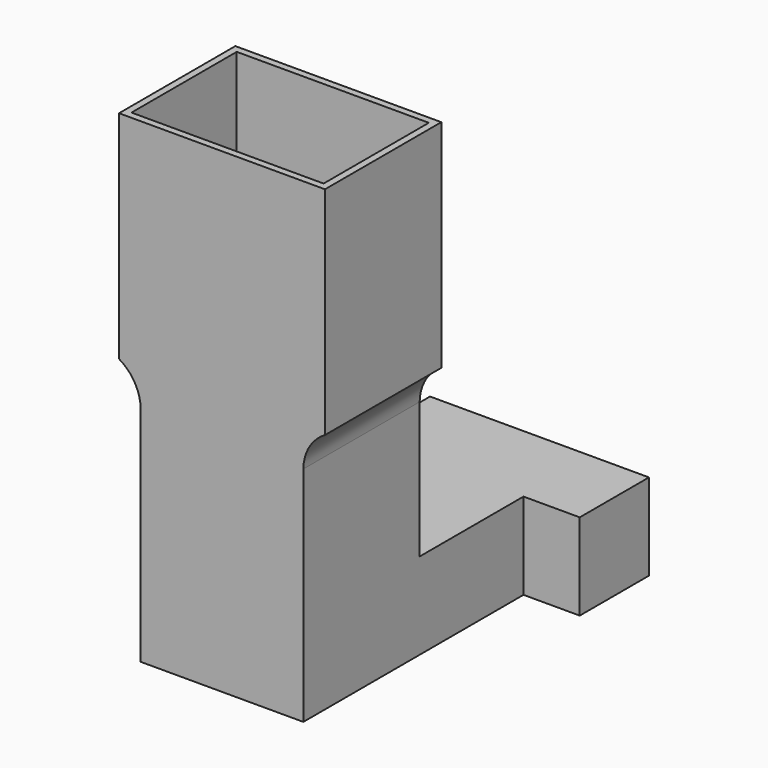
from build123d import *

# Parameters (mm, degrees)
F2_W        = 18.8
F2_H        = 30
F3_DEPTH    = 16.8
F4_T1_DEPTH = 16.8
F5_T        = 0.8
F5_T3_DEPTH = 18.4
F6_W        = 18.8
F6_H        = 10
F7_DEPTH    = 25
F8_T        = -0.8
F9_DEPTH    = 0.8
F10_W       = 0.8
F10_H       = 8.4
F11_DEPTH   = 25.8
F12_W       = 10
F12_H       = 10
F13_DEPTH   = 6.5


# Not quite as in the source:
# - a fillet or chamfer that OpenCascade refuses, or shapes differently, is made with other operations: its cross-section is extruded or revolved along the edge and cut away or added
# - a shell that OpenCascade refuses in one call is made with other operations: the cavity is built on its own and cut out


with BuildPart() as f3:
    # F2 (on Front) → F3 (new body)
    with BuildSketch(Plane.XZ):
        Polygon((23.8, 25), (0, 25), (0, 0), (2.5, 0), (21.3, 0), (23.8, 0), align=None)
        with Locations((11.9, -15)):
            Rectangle(F2_W, F2_H)
    extrude(amount=F3_DEPTH)

    # F4: fillet of radius 5 on 2 edges, made by hand

    # F4_s2 → F4_t1 (join)
    with BuildSketch(Plane.XZ):
        with BuildLine():
            ThreePointArc((0.0002000386, 0.0003463879), (1.8304834454, -1.8302431314), (2.5004, -4.3306845218))
            Line((2.5004, -4.3306845218), (3.0005365685, -4.3306845218))
            ThreePointArc((3.0005365685, -4.3306845218), (3.0001365685, -2.1653422609), (3.0001365685, 0))
            Line((3.0001365685, 0), (2.5, 0.5001365685))
            ThreePointArc((2.5, 0.5001365685), (1.2501000193, 0.5001365685), (0.250316611, 0.4334494788))
            Line((0.250316611, 0.4334494788), (0.0002000386, 0.0003463879))
        make_face()
        with BuildLine():
            ThreePointArc((21.2996, -4.3306845218), (21.9695165546, -1.8302431314), (23.7997999614, 0.0003463879))
            Line((23.7997999614, 0.0003463879), (23.549683389, 0.4334494788))
            ThreePointArc((23.549683389, 0.4334494788), (22.5498999807, 0.5001365685), (21.3, 0.5001365685))
            Line((21.3, 0.5001365685), (20.7998634315, 0))
            ThreePointArc((20.7998634315, 0), (20.7998634315, -2.1653422609), (20.7994634315, -4.3306845218))
            Line((20.7994634315, -4.3306845218), (21.2996, -4.3306845218))
        make_face()
    extrude(amount=F4_T1_DEPTH)

    # F5: shell of thickness 0.8, made by hand


with BuildPart() as f5_core1:
    # F5_t2: copy of F3
    add(f3.part)

    # the walls: a layer under each face that stays
    f5_faces = [f5_core1.faces().sort_by_distance(p)[0] for p in [
        (23.8, -8.4, 12.5),
        (0, -8.4, 12.5),
        (11.9, 0, -2.5),
        (11.9, -16.8, -2.5),
        (23.7996001251, -8.4, 0),
        (0.0003998749, -8.4, 0),
        (21.3, -8.4, -17.1337157982),
        (11.9, -8.4, -30),
        (2.5, -8.4, -17.1337157982),
        (21.9852401758, -8.4, -1.8032011796),
        (1.8147598242, -8.4, -1.8032011796),
    ]]
    thicken(f5_faces, amount=-F5_T, mode=Mode.SUBTRACT)

    # F5_s4 → F5_t3 (cut)
    with BuildSketch(Plane.XZ.offset(-0.8)):
        Polygon((23.803201982, -0.0149272032), (23.7992002503, 0.8), (23.5847337286, 0.8), (23.3990270828, 0.6927203159), align=None)
        Polygon((-0.003201982, -0.0149272032), (0.0007997497, 0.8), (0.2152662714, 0.8), (0.4009729172, 0.6927203159), align=None)
        Polygon((21.3159993602, -4.2675327735), (20.5, -4.2674315965), (20.5, -4.2623725419), (20.5000639825, -4.257313892), align=None)
        Polygon((2.4840006398, -4.2675327735), (3.3, -4.2674315965), (3.3, -4.2623725419), (3.2999360175, -4.257313892), align=None)
    extrude(amount=F5_T3_DEPTH, mode=Mode.SUBTRACT)


with BuildPart() as f3_1:
    add(f3.part)

    # what is left inside the walls is the cavity
    f5_cavity = [f5_core1.part.solids().sort_by_distance(p)[0] for p in [
        (11.9, -15.992, -11.133333),
    ]]
    add(f5_cavity, mode=Mode.SUBTRACT)

    # F6 (on face) → F7 (join)
    with BuildSketch(Plane(origin=(0, 0, 0), x_dir=(-1, 0, 0), z_dir=(0, 1, 0))):
        with Locations((-11.9, -25)):
            Rectangle(F6_W, F6_H)
    extrude(amount=F7_DEPTH)

    # F8
    f8_openings = [f3_1.faces().sort_by_distance(p)[0] for p in [
        (11.9, 25, -25),
    ]]
    offset(amount=F8_T, openings=f8_openings, kind=Kind.INTERSECTION)

    # F9 (cut, through all): a face of the model
    f9_faces = [f3_1.faces().sort_by_distance(p)[0] for p in [
        (11.9, 0, -25),
    ]]
    extrude(f9_faces, amount=-F9_DEPTH, mode=Mode.SUBTRACT)

    # F10 (on face) → F11 (join, through all)
    with BuildSketch(Plane(origin=(0, 25, 0), x_dir=(-1, 0, 0), z_dir=(0, 1, 0))):
        with Locations((-11.9, -25)):
            Rectangle(F10_W, F10_H)
    extrude(amount=-F11_DEPTH)

    # F12 (on face) → F13 (join)
    with BuildSketch(Plane.YZ.offset(21.3)):
        with Locations((20, -25)):
            Rectangle(F12_W, F12_H)
    extrude(amount=F13_DEPTH)


solid = f3_1.part
